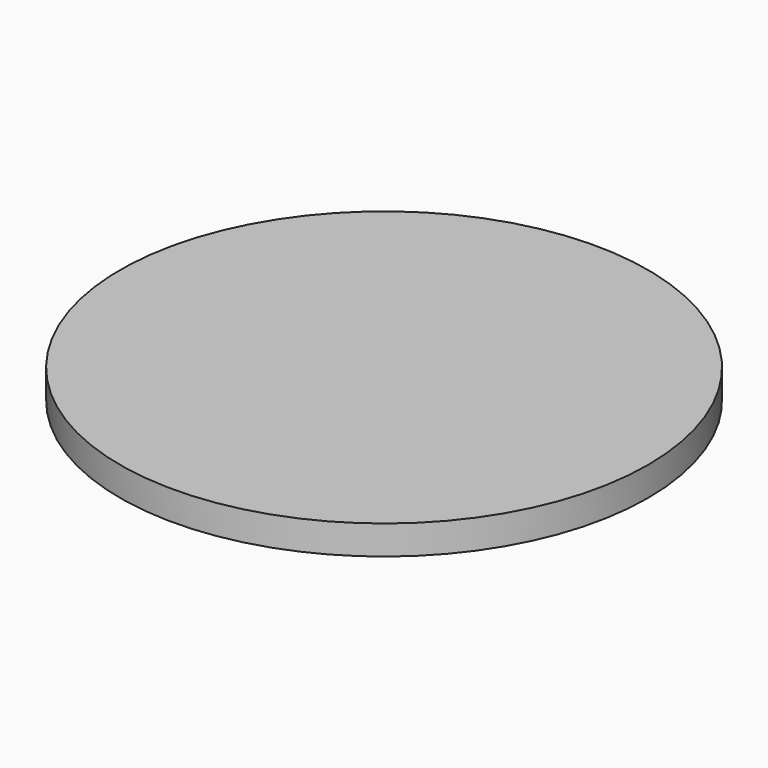
from build123d import *

# Parameters (mm, degrees)
F0_R         = 72.5
F1_DEPTH     = 8
F4_DEPTH     = 0.508
F3_TEXT_SIZE = 8.9035517295
F5_DEPTH     = 6


# Not quite as in the source:
# - Text() gives the source's letters only with a copy of the font that has no kerning and outlines rounded to 1/6400 em; it was checked with that copy


with BuildPart() as f1:
    # F0 (on Top) → F1 (new body)
    with BuildSketch(Plane.XY):
        Circle(F0_R)
    extrude(amount=F1_DEPTH)

    # F0 (on Top) → F4 (cut)
    with BuildSketch(Plane.XY):
        Circle(F0_R)
    extrude(amount=-F4_DEPTH, mode=Mode.SUBTRACT)

    # F3 (on Top) → F5 (cut)
    with BuildSketch(Plane.XY):
        with Locations((-52.4076003236, -4.1520285933)):
            Text('The College of New Jersey', F3_TEXT_SIZE, font='Arimo', font_style=FontStyle.ITALIC, text_align=(TextAlign.LEFT, TextAlign.BOTTOM))
    extrude(amount=-F5_DEPTH, mode=Mode.SUBTRACT)


solid = f1.part
